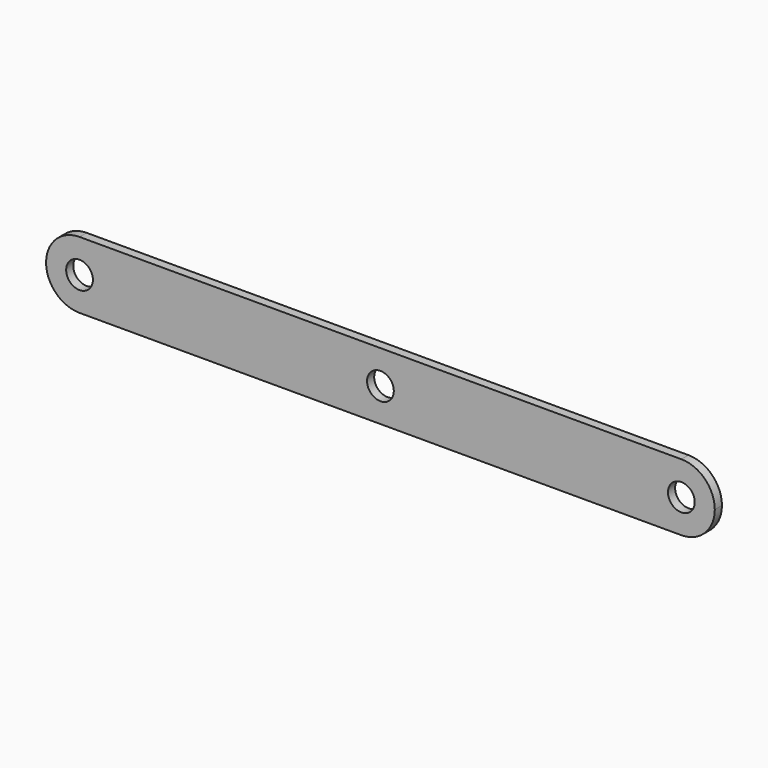
from build123d import *

# Parameters (mm, degrees)
F0_W     = 150
F0_H     = 15
F0_R     = 3
F1_DEPTH = 1
F2_R     = 7.49999


# Not quite as in the source:
# - a fillet or chamfer is up to 0.001 mm smaller than in the source, because OpenCascade refuses the exact size


with BuildPart() as f1:
    # F0 (on Front) → F1 (new body, symmetric)
    with BuildSketch(Plane.XZ):
        with Locations((67.5, 0)):
            Rectangle(F0_W, F0_H)
        Circle(F0_R, mode=Mode.SUBTRACT)
        with Locations((67.5, 0)):
            Circle(F0_R, mode=Mode.SUBTRACT)
        with Locations((135, 0)):
            Circle(F0_R, mode=Mode.SUBTRACT)
    extrude(amount=F1_DEPTH, both=True)

    # F2 (radius 7.5 in the source; OpenCascade refuses exactly that, so slightly less here)
    f2_edges = [f1.edges().sort_by_distance(p)[0] for p in [
        (142.5, 0, 7.5),
        (142.5, 0, -7.5),
        (-7.5, 0, 7.5),
        (-7.5, 0, -7.5),
    ]]
    fillet(f2_edges, radius=F2_R)


solid = f1.part
